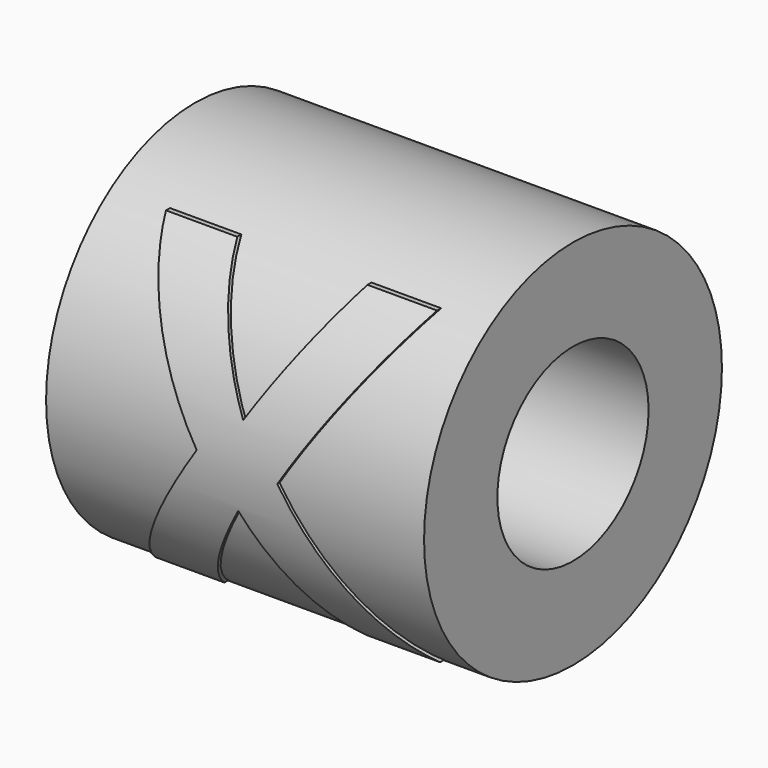
from build123d import *

# Parameters (mm, degrees)
F0_R         = 1
F0_R_2       = 0.985
F0_R_3       = 0.5
F1_DEPTH     = 2
F2_TEXT_SIZE = 2.2604994431
F3_REACH     = 3.2095817879
F4_DEPTH     = 2


# Not quite as in the source:
# - Text() gives the source's letters only with a copy of the font that has no kerning and outlines rounded to 1/6400 em; it was checked with that copy


with BuildPart() as f1:
    # F0 (on Right) → F1 (new body)
    with BuildSketch(Plane.YZ):
        Circle(F0_R)
        Circle(F0_R_2, mode=Mode.SUBTRACT)
        Circle(F0_R_2)
        Circle(F0_R_3, mode=Mode.SUBTRACT)
    extrude(amount=F1_DEPTH)

    f3_end = f1.faces().sort_by_distance((1, -1, 0))[0]
    # F2 (on Front) → F3 (intersect, up to a face of the model that its end follows)
    with BuildSketch(Plane.XZ):
        with Locations((0.2728080435, -0.7963191019)):
            Text('X', F2_TEXT_SIZE, font='Open Sans', font_style=FontStyle.BOLD, text_align=(TextAlign.LEFT, TextAlign.BOTTOM))
    f3_long = extrude(amount=F3_REACH, mode=Mode.PRIVATE)
    add(split(f3_long, bisect_by=f3_end, keep=Keep.BOTTOM, mode=Mode.PRIVATE), mode=Mode.INTERSECT)


with BuildPart() as f4:
    # F0 (on Right) → F4 (new body)
    with BuildSketch(Plane.YZ):
        Circle(F0_R_2)
        Circle(F0_R_3, mode=Mode.SUBTRACT)
    extrude(amount=F4_DEPTH)


solid = Compound([f1.part, f4.part])
